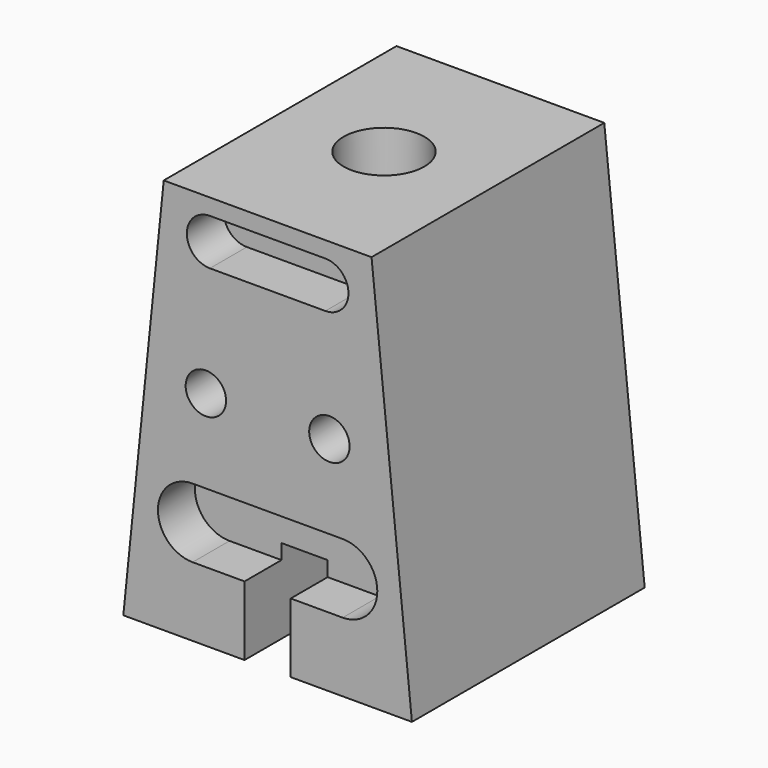
from build123d import *

# Parameters (mm, degrees)
F0_R           = 0.875
F1_DEPTH       = 12.6
F2_DEPTH       = 2
F4_D           = 2
F4_DEPTH       = 38
F4_CBORE_D     = 3.5
F4_CBORE_DEPTH = 3
F4_TIP         = 0.600860619


# Not quite as in the source:
# - a feature names something its author has since deleted; it is built from what else it names


with BuildPart() as f1:
    # F0 (on Front) → F1 (new body)
    with BuildSketch(Plane.XZ):
        with BuildLine():
            Line((1, 0), (6.25, 0))
            Line((6.25, 0), (4.5, 17.15))
            Line((4.5, 17.15), (0, 17.15))
            Line((0, 17.15), (-4.5, 17.15))
            Line((-4.5, 17.15), (-6.25, 0))
            Line((-6.25, 0), (-1, 0))
            Line((-1, 0), (-1, 3))
            Line((-1, 3), (-3.25, 3))
            ThreePointArc((-3.25, 3), (-4.75, 4.5), (-3.25, 6))
            Line((-3.25, 6), (0, 6))
            Line((0, 6), (3.25, 6))
            ThreePointArc((3.25, 6), (4.75, 4.5), (3.25, 3))
            Line((3.25, 3), (1, 3))
            Line((1, 3), (1, 0))
        make_face()
        with Locations((-2.675, 9.625)):
            Circle(F0_R, mode=Mode.SUBTRACT)
        with Locations((2.675, 9.625)):
            Circle(F0_R, mode=Mode.SUBTRACT)
        with BuildLine():
            Line((-2.5, 16.4487531745), (0, 16.4487531745))
            Line((0, 16.4487531745), (2.5, 16.4487531745))
            ThreePointArc((2.5, 16.4487531745), (3.5, 15.4487531745), (2.5, 14.4487531745))
            Line((2.5, 14.4487531745), (0, 14.4487531745))
            Line((0, 14.4487531745), (-2.5, 14.4487531745))
            ThreePointArc((-2.5, 14.4487531745), (-3.5, 15.4487531745), (-2.5, 16.4487531745))
        make_face(mode=Mode.SUBTRACT)
        with BuildLine():
            Line((2.5, 16.4487531745), (0, 16.4487531745))
            Line((0, 16.4487531745), (-2.5, 16.4487531745))
            ThreePointArc((-2.5, 16.4487531745), (-3.5, 15.4487531745), (-2.5, 14.4487531745))
            Line((-2.5, 14.4487531745), (0, 14.4487531745))
            Line((0, 14.4487531745), (2.5, 14.4487531745))
            ThreePointArc((2.5, 14.4487531745), (3.5, 15.4487531745), (2.5, 16.4487531745))
        make_face()
        with Locations((-2.675, 9.625)):
            Circle(F0_R)
        with Locations((2.675, 9.625)):
            Circle(F0_R)
        with BuildLine():
            Line((1, 3.65), (1, 3))
            Line((1, 3), (3.25, 3))
            ThreePointArc((3.25, 3), (4.75, 4.5), (3.25, 6))
            Line((3.25, 6), (0, 6))
            Line((0, 6), (-3.25, 6))
            ThreePointArc((-3.25, 6), (-4.75, 4.5), (-3.25, 3))
            Line((-3.25, 3), (-1, 3))
            Line((-1, 3), (-1, 3.65))
            Line((-1, 3.65), (0, 3.65))
            Line((0, 3.65), (1, 3.65))
        make_face()
    extrude(amount=-F1_DEPTH)

    # F0 (on Front) → F2 (cut)
    with BuildSketch(Plane.XZ):
        with BuildLine():
            Line((1, 3.65), (1, 3))
            Line((1, 3), (3.25, 3))
            ThreePointArc((3.25, 3), (4.75, 4.5), (3.25, 6))
            Line((3.25, 6), (0, 6))
            Line((0, 6), (-3.25, 6))
            ThreePointArc((-3.25, 6), (-4.75, 4.5), (-3.25, 3))
            Line((-3.25, 3), (-1, 3))
            Line((-1, 3), (-1, 3.65))
            Line((-1, 3.65), (0, 3.65))
            Line((0, 3.65), (1, 3.65))
        make_face()
        with BuildLine():
            Line((2.5, 16.4487531745), (0, 16.4487531745))
            Line((0, 16.4487531745), (-2.5, 16.4487531745))
            ThreePointArc((-2.5, 16.4487531745), (-3.5, 15.4487531745), (-2.5, 14.4487531745))
            Line((-2.5, 14.4487531745), (0, 14.4487531745))
            Line((0, 14.4487531745), (2.5, 14.4487531745))
            ThreePointArc((2.5, 14.4487531745), (3.5, 15.4487531745), (2.5, 16.4487531745))
        make_face()
        with Locations((2.675, 9.625)):
            Circle(F0_R)
        with Locations((-2.675, 9.625)):
            Circle(F0_R)
    extrude(amount=-F2_DEPTH, mode=Mode.SUBTRACT)

    # F4
    with Locations(Plane.XY.offset(17.15)):
        with Locations((0, 6.3)):
            CounterBoreHole(F4_D / 2, F4_CBORE_D / 2, F4_CBORE_DEPTH, depth=F4_DEPTH)
            with Locations((0, 0, -(F4_DEPTH + F4_TIP / 2))):  # 118° drill point
                Cone(0, F4_D / 2, F4_TIP, mode=Mode.SUBTRACT)


solid = f1.part
